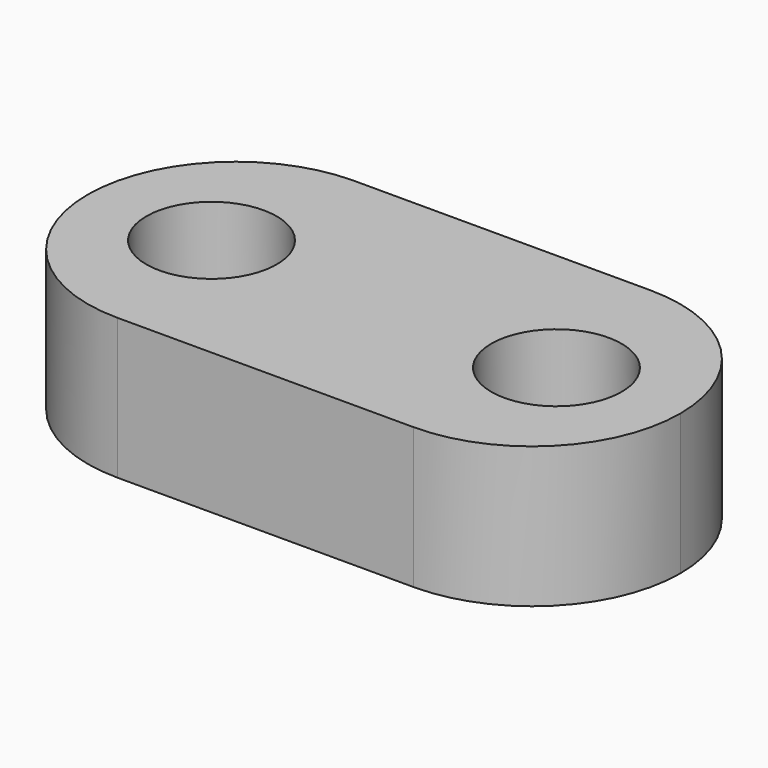
from build123d import *

# Parameters (mm, degrees)
F0_W     = 20
F0_H     = 10
F1_DEPTH = 4.75
F2_D     = 4.4
F2_DEPTH = 25
F2_TIP   = 1.3218933619
F3_R     = 4.99999


# Not quite as in the source:
# - a fillet or chamfer is up to 0.001 mm smaller than in the source, because OpenCascade refuses the exact size


with BuildPart() as f1:
    # F0 (on Top) → F1 (new body)
    with BuildSketch(Plane.XY):
        Rectangle(F0_W, F0_H)
    extrude(amount=F1_DEPTH)

    # F2
    with Locations(Plane(origin=(0, 0, 0), x_dir=(1, 0, 0), z_dir=(0, 0, -1))):
        with Locations((-5.82, 0), (5.82, 0)):
            Hole(F2_D / 2, depth=F2_DEPTH)
            with Locations((0, 0, -(F2_DEPTH + F2_TIP / 2))):  # 118° drill point
                Cone(0, F2_D / 2, F2_TIP, mode=Mode.SUBTRACT)

    # F3 (radius 5 in the source; OpenCascade refuses exactly that, so slightly less here)
    f3_edges = [f1.edges().sort_by_distance(p)[0] for p in [
        (10, 5, 2.375),
        (10, -5, 2.375),
        (-10, 5, 2.375),
        (-10, -5, 2.375),
    ]]
    fillet(f3_edges, radius=F3_R)


solid = f1.part
